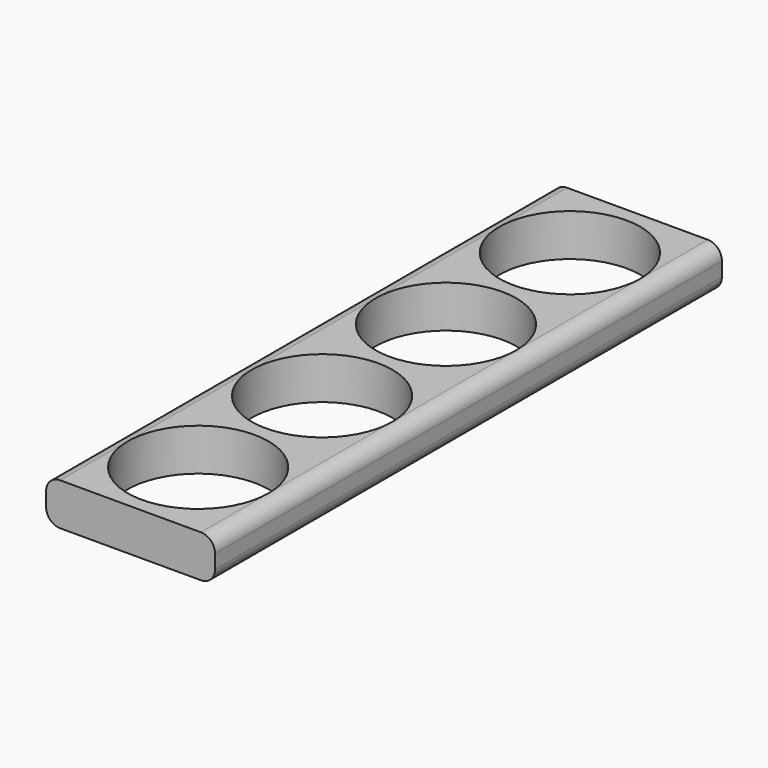
from build123d import *

# Parameters (mm, degrees)
F0_W     = 12
F0_H     = 45
F0_R     = 5
F1_DEPTH = 3
F2_R     = 0.99999


# Not quite as in the source:
# - a fillet or chamfer is up to 0.001 mm smaller than in the source, because OpenCascade refuses the exact size


with BuildPart() as f1:
    # F0 (on Top) → F1 (new body)
    with BuildSketch(Plane.XY):
        with Locations((6, 22.5)):
            Rectangle(F0_W, F0_H)
        with Locations((6, 6)):
            Circle(F0_R, mode=Mode.SUBTRACT)
        with Locations((6, 17)):
            Circle(F0_R, mode=Mode.SUBTRACT)
        with Locations((6, 28)):
            Circle(F0_R, mode=Mode.SUBTRACT)
        with Locations((6, 39)):
            Circle(F0_R, mode=Mode.SUBTRACT)
    extrude(amount=F1_DEPTH)

    # F2 (radius 1 in the source; OpenCascade refuses exactly that, so slightly less here)
    f2_edges = [f1.edges().sort_by_distance(p)[0] for p in [
        (12, 22.5, 3),
        (12, 22.5, 0),
        (0, 22.5, 3),
        (0, 22.5, 0),
    ]]
    fillet(f2_edges, radius=F2_R)


solid = f1.part
